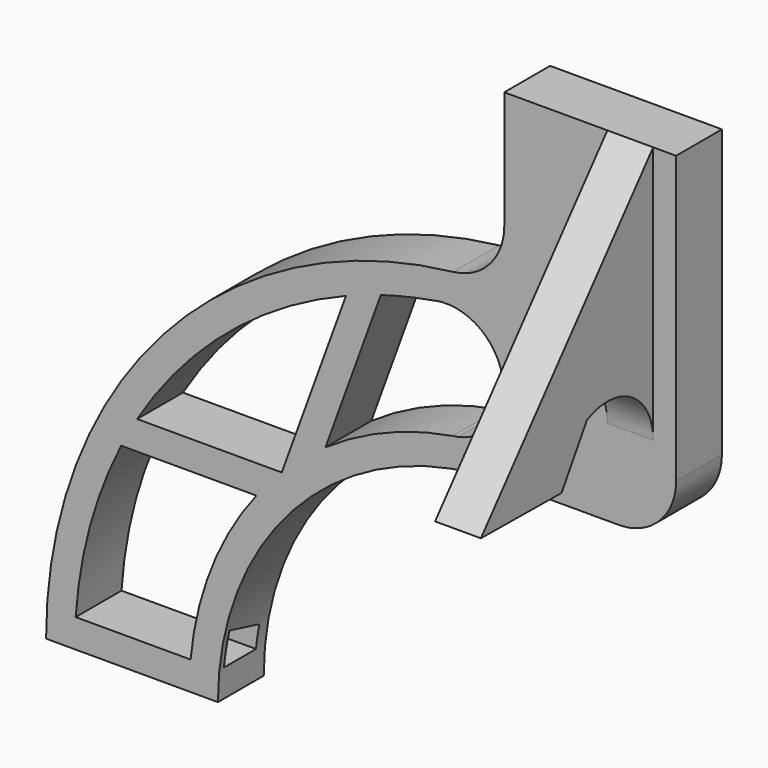
from build123d import *

# Parameters (mm, degrees)
F1_DEPTH = 10
F2_R     = 10
F4_DEPTH = 55
F6_START = -4
F6_DEPTH = 8


# Not quite as in the source:
# - a feature names something its author has since deleted; it is built from what else it names


with BuildPart() as f1:
    # F0 (on Front) → F1 (new body)
    with BuildSketch(Plane.XZ):
        with BuildLine():
            ThreePointArc((-50, 0), (-35.3553390593, 35.3553390593), (0, 50))
            Line((0, 50), (30, 50))
            Line((30, 50), (30, 110))
            Line((30, 110), (0, 110))
            Line((0, 110), (0, 89.4427191))
            ThreePointArc((0, 89.4427191), (-2.546440075, 82.7760524333), (-8.8888888889, 79.5046392))
            ThreePointArc((-8.8888888889, 79.5046392), (-59.6284794, 53.3333333333), (-80, 0))
            Line((-80, 0), (-50, 0))
        make_face()
        with BuildLine():
            Line((-0.1396715456, 63.5967118692), (-0.0513620047, 54.9999760177))
            ThreePointArc((-0.0513620047, 54.9999760177), (-4.1045972669, 54.8466250673), (-8.135508632, 54.3949767837))
            ThreePointArc((-8.135508632, 54.3949767837), (-8.5642581923, 54.317769449), (-8.9959636029, 54.2593092368))
            ThreePointArc((-8.9959636029, 54.2593092368), (-20.6018520556, 50.99572229), (-31.2178460585, 45.2818516347))
            ThreePointArc((-31.2178460585, 45.2818516347), (-35.1775050235, 42.2793464983), (-38.85, 38.9317030195))
            ThreePointArc((-38.85, 38.9317030195), (-41.1438023454, 36.4991442169), (-43.2855579864, 33.9317030195))
            ThreePointArc((-43.2855579864, 33.9317030195), (-51.1184366801, 20.2954534658), (-54.7722557505, 5))
            Line((-54.7722557505, 5), (-74.8331477355, 5))
            ThreePointArc((-74.8331477355, 5), (-72.3207331298, 19.8673490824), (-66.8852713996, 33.9317030195))
            ThreePointArc((-66.8852713996, 33.9317030195), (-65.5423309322, 36.4582344057), (-64.1039975353, 38.9317030195))
            ThreePointArc((-64.1039975353, 38.9317030195), (-48.3880483763, 57.3026768513), (-27.6441832414, 69.7194315304))
            ThreePointArc((-27.6441832414, 69.7194315304), (-24.6212334453, 70.8434532164), (-21.5527545012, 71.8364724455))
            ThreePointArc((-21.5527545012, 71.8364724455), (-17.0660687419, 73.0325221918), (-12.5139679551, 73.9486349165))
            ThreePointArc((-12.5139679551, 73.9486349165), (-11.6819966677, 74.1162256952), (-10.8388112367, 74.2126685343))
            ThreePointArc((-10.8388112367, 74.2126685343), (-5.5617429138, 74.7934958119), (-0.2568067386, 74.999560334))
            Line((-0.2568067386, 74.999560334), (-0.1540837044, 64.9997032265))
            ThreePointArc((-0.1540837044, 64.9997032265), (-0.1222411681, 64.2984606247), (-0.1396715456, 63.5967118692))
        make_face(mode=Mode.SUBTRACT)
        with BuildLine():
            ThreePointArc((-38.85, 38.9317030195), (-35.1775050235, 42.2793464983), (-31.2178460585, 45.2818516347))
            Line((-31.2178460585, 45.2818516347), (-21.5527545012, 71.8364724455))
            ThreePointArc((-21.5527545012, 71.8364724455), (-24.6212334453, 70.8434532164), (-27.6441832414, 69.7194315304))
            Line((-27.6441832414, 69.7194315304), (-38.85, 38.9317030195))
        make_face()
        with BuildLine():
            ThreePointArc((-43.2855579864, 33.9317030195), (-41.1438023454, 36.4991442169), (-38.85, 38.9317030195))
            Line((-38.85, 38.9317030195), (-64.1039975353, 38.9317030195))
            ThreePointArc((-64.1039975353, 38.9317030195), (-65.5423309322, 36.4582344057), (-66.8852713996, 33.9317030195))
            Line((-66.8852713996, 33.9317030195), (-43.2855579864, 33.9317030195))
        make_face()
        with BuildLine():
            ThreePointArc((-10.8388112367, 74.2126685343), (-3.5948385174, 71.8115750097), (-0.1540837044, 64.9997032265))
            Line((-0.1540837044, 64.9997032265), (-0.2568067386, 74.999560334))
            ThreePointArc((-0.2568067386, 74.999560334), (-5.5617429138, 74.7934958119), (-10.8388112367, 74.2126685343))
        make_face()
        with BuildLine():
            ThreePointArc((-8.135508632, 54.3949767837), (-4.1045972669, 54.8466250673), (-0.0513620047, 54.9999760177))
            Line((-0.0513620047, 54.9999760177), (-0.1396715456, 63.5967118692))
            ThreePointArc((-0.1396715456, 63.5967118692), (-2.5733550789, 57.6366041193), (-8.135508632, 54.3949767837))
        make_face()
    extrude(amount=F1_DEPTH)

    # F2
    f2_edges = [f1.edges().sort_by_distance(p)[0] for p in [
        (30, -5, 50),
    ]]
    fillet(f2_edges, radius=F2_R)

    # F3 (on Right) → F4 (cut)
    with BuildSketch(Plane.YZ):
        Polygon((-9, 11), (-9, 5), (-2, 5), (-2, 9), align=None)
    extrude(amount=-F4_DEPTH, mode=Mode.SUBTRACT)

    # F5 (on face) → F6 (join)
    with BuildSketch(Plane.YZ.offset(30).offset(F6_START)):
        with BuildLine():
            Line((-10, 65), (-10, 110))
            Line((-10, 110), (-47.6030751667, 65.1864000775))
            Line((-47.6030751667, 65.1864000775), (-30, 65))
            ThreePointArc((-30, 65), (-28.5022679561, 70.2641656131), (-24.4577120796, 73.9514693216))
            ThreePointArc((-24.4577120796, 73.9514693216), (-14.7358343869, 73.5022679561), (-10, 65))
        make_face()
        with BuildLine():
            ThreePointArc((-24.4577120796, 73.9514693216), (-28.5022679561, 70.2641656131), (-30, 65))
            add(Edge.make_bspline(
                [(-24.4577120796, 73.9514693216), (-26.3063166684, 70.9700062817), (-28.1513954112, 67.9814630399), (-30, 65)],
                knots=[0, 0, 0, 0, 10.5283312262, 10.5283312262, 10.5283312262, 10.5283312262], degree=3))
        make_face()
    extrude(amount=-F6_DEPTH)


solid = f1.part
